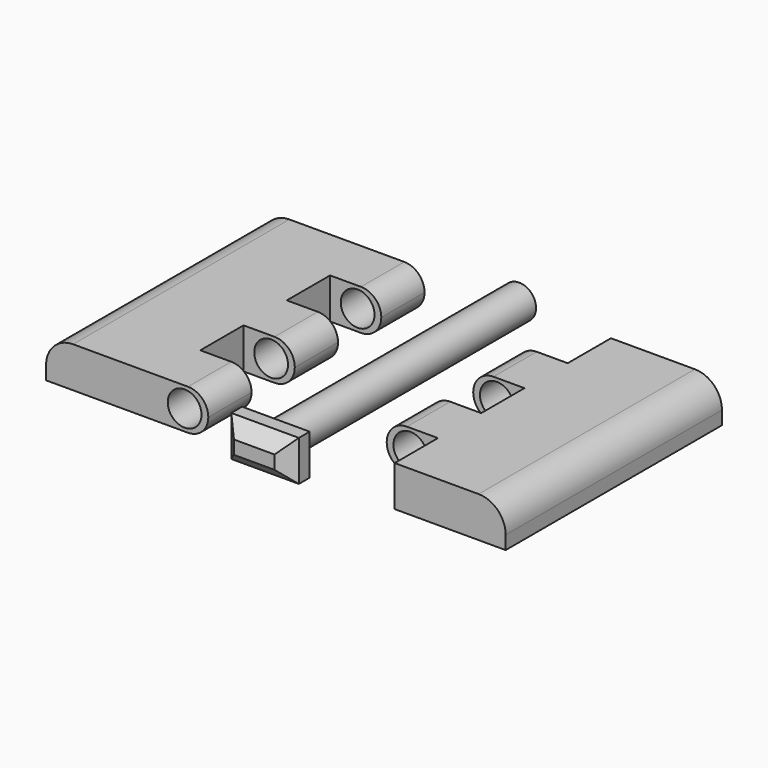
from build123d import *

# Parameters (mm, degrees)
F0_W      = 30.48
F0_H      = 50.8
F1_DEPTH  = 7.62
F2_R      = 3.175
F3_DEPTH  = 50.8
F4_W      = 9.6290465444
F4_H      = 10.16
F5_DEPTH  = 7.62
F6_DEPTH  = 7.62
F7_R      = 5.08
F7_2_R    = 5.08
F8_R      = 3.80999
F8_2_R    = 3.80999
F9_W      = 12.7
F9_H      = 7.62
F9_R      = 3.175
F10_DEPTH = 5.08
F11_DEPTH = 57.15
F12_SIZE  = 2.54


# Not quite as in the source:
# - a fillet or chamfer is up to 0.001 mm smaller than in the source, because OpenCascade refuses the exact size


with BuildPart() as f1:
    # F0 (on Top) → F1 (new body)
    with BuildSketch(Plane.XY):
        with Locations((15.24, 25.4)):
            Rectangle(F0_W, F0_H)
    extrude(amount=F1_DEPTH)


with BuildPart() as f1b:
    # F0 (on Top) → F1, piece 2 (new body)
    with BuildSketch(Plane.XY):
        with Locations((-40.64, 25.4)):
            Rectangle(F0_W, F0_H)
    extrude(amount=F1_DEPTH)


with BuildPart() as f3_tool:
    # F2 (on face) → F3 (new body, through all)
    with BuildSketch(Plane.XZ):
        with Locations((4.445, 3.81)):
            Circle(F2_R)
        with Locations((-29.845, 3.81)):
            Circle(F2_R)
    extrude(amount=-F3_DEPTH)


with BuildPart() as f1_1:
    add(f1.part)

    # F3: cut by f3_tool
    add(f3_tool.part, mode=Mode.SUBTRACT)

    # F4 (on face) → F5 (cut, through all)
    with BuildSketch(Plane.XY.offset(7.62)):
        with Locations((4.8145232722, 5.08)):
            Rectangle(F4_W, F4_H)
        with Locations((4.8145232722, 25.4)):
            Rectangle(F4_W, F4_H)
        with Locations((4.8145232722, 45.72)):
            Rectangle(F4_W, F4_H)
    extrude(amount=-F5_DEPTH, mode=Mode.SUBTRACT)

    # F7#2
    f7_2_edges = [f1_1.edges().sort_by_distance(p)[0] for p in [
        (30.48, 25.4, 7.62),
    ]]
    fillet(f7_2_edges, radius=F7_2_R)

    # F8 (radius 3.81 in the source; OpenCascade refuses exactly that, so slightly less here)
    f8_edges = [f1_1.edges().sort_by_distance(p)[0] for p in [
        (0, 15.24, 7.62),
        (0, 15.24, 0),
        (0, 35.56, 7.62),
        (0, 35.56, 0),
    ]]
    fillet(f8_edges, radius=F8_R)


with BuildPart() as f1b_1:
    add(f1b.part)

    # F3: cut by f3_tool
    add(f3_tool.part, mode=Mode.SUBTRACT)

    # F4 (on face) → F6 (cut, through all)
    with BuildSketch(Plane.XY.offset(7.62)):
        with Locations((-30.2145232722, 15.24)):
            Rectangle(F4_W, F4_H)
        with Locations((-30.2145232722, 35.56)):
            Rectangle(F4_W, F4_H)
    extrude(amount=-F6_DEPTH, mode=Mode.SUBTRACT)

    # F7
    f7_edges = [f1b_1.edges().sort_by_distance(p)[0] for p in [
        (-55.88, 25.4, 7.62),
    ]]
    fillet(f7_edges, radius=F7_R)

    # F8#2 (radius 3.81 in the source; OpenCascade refuses exactly that, so slightly less here)
    f8_2_edges = [f1b_1.edges().sort_by_distance(p)[0] for p in [
        (-25.4, 5.08, 0),
        (-25.4, 5.08, 7.62),
        (-25.4, 25.4, 0),
        (-25.4, 25.4, 7.62),
        (-25.4, 45.72, 0),
        (-25.4, 45.72, 7.62),
    ]]
    fillet(f8_2_edges, radius=F8_2_R)


with BuildPart() as f10:
    # F9 (on face) → F10 (new body)
    with BuildSketch(Plane.XZ):
        with Locations((-12.7, 3.81)):
            Rectangle(F9_W, F9_H)
        with Locations((-12.7, 3.81)):
            Circle(F9_R, mode=Mode.SUBTRACT)
        with Locations((-12.7, 3.81)):
            Circle(F9_R)
    extrude(amount=F10_DEPTH)

    # F9 (on face) → F11 (join)
    with BuildSketch(Plane.XZ):
        with Locations((-12.7, 3.81)):
            Circle(F9_R)
    extrude(amount=-F11_DEPTH)

    # F12
    f12_edges = [f10.edges().sort_by_distance(p)[0] for p in [
        (-6.35, -5.08, 3.81),
        (-12.7, -5.08, 7.62),
        (-19.05, -5.08, 3.81),
        (-12.7, -5.08, 0),
    ]]
    chamfer(f12_edges, length=F12_SIZE)


solid = Compound([f1_1.part, f1b_1.part, f10.part])
